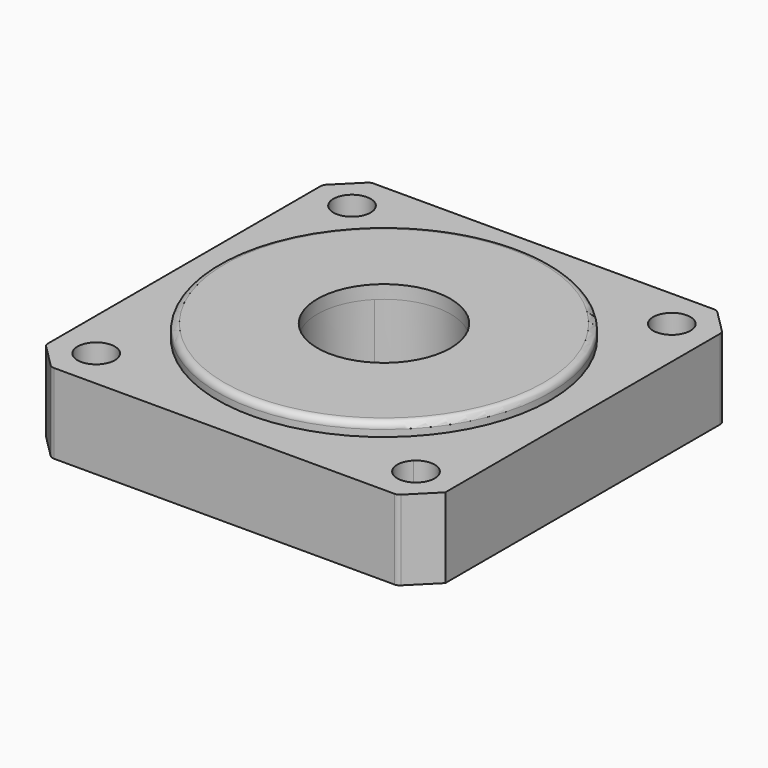
from build123d import *
from build123d import SkipClean  # not in build123d's __all__

# Parameters (mm, degrees)
F1_DEPTH = 7.62
F2_R     = 15.875
F2_R_2   = 6.35
F3_DEPTH = 1.27
F4_R     = 0.635


with BuildPart() as f1:
    # F0 (on Top) → F1 (new body)
    with BuildSketch(Plane.XY):
        Polygon((16.51, 19.05), (-16.51, 19.05), (-19.05, 16.51), (-19.05, -16.51), (-16.51, -19.05), (16.51, -19.05), (19.05, -16.51), (19.05, 0), (19.05, 16.51), align=None)
        with BuildLine():
            ThreePointArc((-13.4704748936, -15.2484748936), (-16.8911327024, -15.9288860363), (-13.9912390366, -13.9912390366))
            ThreePointArc((-13.9912390366, -13.9912390366), (-13.6058170848, -14.5680637508), (-13.4704748936, -15.2484748936))
        make_face(mode=Mode.SUBTRACT)
        with BuildLine():
            ThreePointArc((17.0264748936, -15.2484748936), (14.5680637508, -16.8911327024), (13.9912390366, -13.9912390366))
            ThreePointArc((13.9912390366, -13.9912390366), (15.9288860363, -13.6058170848), (17.0264748936, -15.2484748936))
        make_face(mode=Mode.SUBTRACT)
        with BuildLine():
            ThreePointArc((-13.4704748936, 15.2484748936), (-13.6058170848, 14.5680637508), (-13.9912390366, 13.9912390366))
            ThreePointArc((-13.9912390366, 13.9912390366), (-16.8911327024, 15.9288860363), (-13.4704748936, 15.2484748936))
        make_face(mode=Mode.SUBTRACT)
        with BuildLine():
            ThreePointArc((4.4901280605, 4.4901280605), (5.8666350314, 2.4300397955), (6.35, 0))
            ThreePointArc((6.35, 0), (5.8666350314, -2.4300397955), (4.4901280605, -4.4901280605))
            ThreePointArc((4.4901280605, -4.4901280605), (0, -6.35), (-4.4901280605, -4.4901280605))
            ThreePointArc((-4.4901280605, -4.4901280605), (-6.35, 0), (-4.4901280605, 4.4901280605))
            ThreePointArc((-4.4901280605, 4.4901280605), (0, 6.35), (4.4901280605, 4.4901280605))
        make_face(mode=Mode.SUBTRACT)
        with BuildLine():
            ThreePointArc((17.0264748936, 15.2484748936), (15.9288860363, 13.6058170848), (13.9912390366, 13.9912390366))
            ThreePointArc((13.9912390366, 13.9912390366), (14.5680637508, 16.8911327024), (17.0264748936, 15.2484748936))
        make_face(mode=Mode.SUBTRACT)
    extrude(amount=F1_DEPTH)

    # F2 (on face) → F3 (join)
    with BuildSketch(Plane.XY.offset(7.62)):
        Circle(F2_R)
        Circle(F2_R_2, mode=Mode.SUBTRACT)
    with SkipClean():  # cleaning this boolean's faces spoils the solid; the shape is the same uncleaned
        extrude(amount=F3_DEPTH)

    # F4
    f4_edges = [f1.edges().sort_by_distance(p)[0] for p in [
        (-15.875, 0, 8.89),
        (-19.05, 16.51, 3.81),
        (-19.05, -16.51, 3.81),
        (-16.51, -19.05, 3.81),
        (16.51, -19.05, 3.81),
        (19.05, 16.51, 3.81),
        (16.51, 19.05, 3.81),
        (-16.51, 19.05, 3.81),
    ]]
    fillet(f4_edges, radius=F4_R)


solid = f1.part
